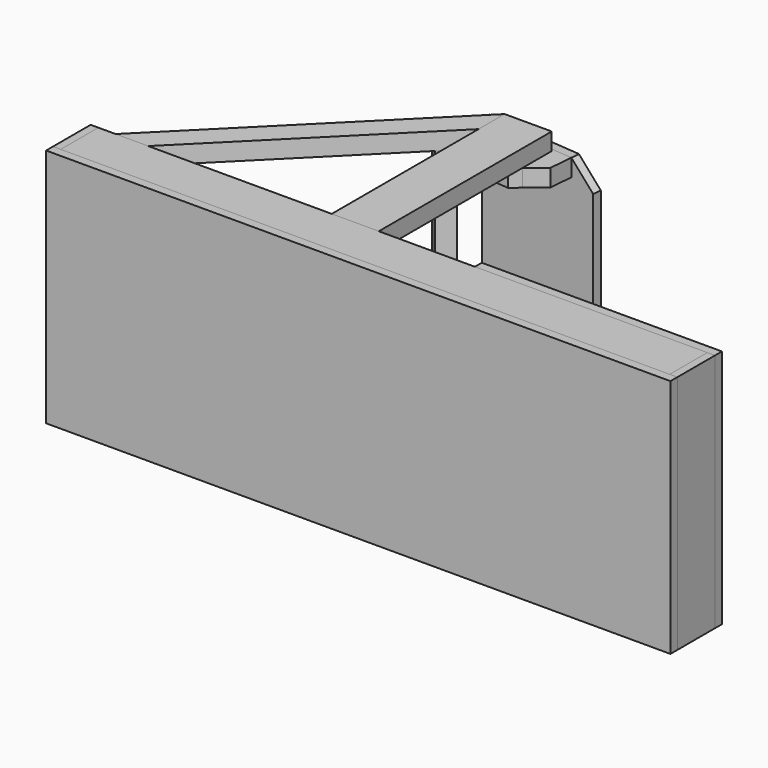
from build123d import *

# Parameters (mm, degrees)
F1_DEPTH       = 500
F2_DEPTH       = 36
F3_DEPTH       = 36
F4_DEPTH       = 36
F5_DEPTH       = 500
F0_W           = 16
F0_H           = 98
F6_DEPTH       = 500
F8_DEPTH       = 36
F9_DEPTH       = 428
F14_W          = 98
F14_H          = 428
F15_DEPTH      = 36
F16_W          = 98
F16_H          = 48
F17_DEPTH      = 36
F16_H_2        = 18
F18_DEPTH      = 104
F18_DEPTH_BACK = 36
F19_W          = 98
F19_H          = 36
F20_DEPTH      = 18
F22_DEPTH      = 36
F24_DEPTH      = 428
F26_DEPTH      = 18


with BuildPart() as f1:
    # F0 (on Top) → F1 (new body)
    with BuildSketch(Plane.XY):
        Polygon((1268, -98), (0, -98), (-16, -98), (-16, -116), (1284, -116), (1284, -98), align=None)
    extrude(amount=-F1_DEPTH)


with BuildPart() as f2:
    # F0 (on Top) → F2 (new body)
    with BuildSketch(Plane.XY):
        Polygon((36, 0), (0, 0), (0, -98), (1268, -98), (1268, 0), (784, 0), (584, 0), (486, 0), (103.8822509939, 0), align=None)
    extrude(amount=-F2_DEPTH)


with BuildPart() as f3:
    # F0 (on Top) → F3 (new body)
    with BuildSketch(Plane.XY):
        Polygon((584, 450), (486, 450), (486, 382.1177490061), (486, 0), (584, 0), align=None)
    extrude(amount=-F3_DEPTH)


with BuildPart() as f4:
    # F0 (on Top) → F4 (new body)
    with BuildSketch(Plane.XY):
        Polygon((486, 450), (36, 0), (103.8822509939, 0), (486, 382.1177490061), align=None)
    extrude(amount=-F4_DEPTH)


with BuildPart() as f5:
    # F0 (on Top) → F5 (new body)
    with BuildSketch(Plane.XY):
        Polygon((784, 0), (1268, 0), (1284, 0), (1284, 18), (784, 18), align=None)
    extrude(amount=-F5_DEPTH)


with BuildPart() as f6:
    # F0 (on Top) → F6 (new body)
    with BuildSketch(Plane.XY):
        with Locations((1276, -49)):
            Rectangle(F0_W, F0_H)
    extrude(amount=-F6_DEPTH)


with BuildPart() as f8:
    # F7 (on face) → F8 (new body)
    with BuildSketch(Plane(origin=(0, 0, -36), x_dir=(1, 0, 0), z_dir=(0, 0, -1))):
        Polygon((418.8753596794, -419.6689985812), (423.2171666194, -469.2960789942), (623.4523009358, -451.7777747019), (619.1816695412, -402.9642344955), (584, -373.4433085592), (584, -450), (486, -450), (486, -365.4289487301), (462.6759038301, -367.469542732), align=None)
        Polygon((566.0974979401, -358.4213256836), (486, -365.4289487301), (486, -450), (584, -450), (584, -373.4433085592), align=None)
    extrude(amount=F8_DEPTH)


with BuildPart() as f9:
    # F7 (on face) → F9 (new body)
    with BuildSketch(Plane(origin=(0, 0, -36), x_dir=(1, 0, 0), z_dir=(0, 0, -1))):
        Polygon((423.2171666194, -469.2960789942), (424.7859699888, -487.2275835599), (673.8346445118, -465.438647873), (672.2658411423, -447.5071433073), (623.4523009358, -451.7777747019), align=None)
    extrude(amount=F9_DEPTH)

    # F25 (on face) → F26 (cut, through all)
    with BuildSketch(Plane(origin=(43.9610143142, 502.4766928934, 0), x_dir=(0.9961946981, -0.0871557427, 0), z_dir=(-0.0871557427, -0.9961946981, 0))):
        Polygon((630.7048491943, -36), (581.7048491943, -36), (630.7048491943, -85), align=None)
        Polygon((630.7048491943, -464), (630.7048491943, -415), (581.7048491943, -464), align=None)
    extrude(amount=-F26_DEPTH, mode=Mode.SUBTRACT)


with BuildPart() as f11_1:
    # F11: instance of F3
    add(f3.part.mirror(Plane(origin=(317, -53.5, -250), x_dir=(1, 0, 0), z_dir=(0, 0, 1))))


with BuildPart() as f11_2:
    # F11: instance of F2
    add(f2.part.mirror(Plane(origin=(317, -53.5, -250), x_dir=(1, 0, 0), z_dir=(0, 0, 1))))


with BuildPart() as f11_3:
    # F11: instance of F4
    add(f4.part.mirror(Plane(origin=(317, -53.5, -250), x_dir=(1, 0, 0), z_dir=(0, 0, 1))))


with BuildPart() as f11_4:
    # F11: instance of F8
    add(f8.part.mirror(Plane(origin=(317, -53.5, -250), x_dir=(1, 0, 0), z_dir=(0, 0, 1))))


with BuildPart() as f13_1:
    # F13: instance of F6
    add(f6.part.mirror(Plane(origin=(634, -107, -250), x_dir=(0, -1, 0), z_dir=(-1, 0, 0))))


with BuildPart() as f15:
    # F14 (on face) → F15 (new body)
    with BuildSketch(Plane(origin=(784, 0, 0), x_dir=(0, -1, 0), z_dir=(-1, 0, 0))):
        with Locations((49, -250)):
            Rectangle(F14_W, F14_H)
    extrude(amount=-F15_DEPTH)


with BuildPart() as f17:
    # F16 (on face) → F17 (new body)
    with BuildSketch(Plane(origin=(0, 0, -500), x_dir=(1, 0, 0), z_dir=(0, 0, -1))):
        with Locations((535, -308)):
            Rectangle(F16_W, F16_H)
        Polygon((368, -332), (486, -332), (486, -284), (320, -284), align=None)
        Polygon((584, -284), (584, -332), (744, -332), (696, -284), align=None)
    extrude(amount=F17_DEPTH)


with BuildPart() as f18:
    # F16 (on face) → F18 (new body, two sides)
    with BuildSketch(Plane(origin=(0, 0, -500), x_dir=(1, 0, 0), z_dir=(0, 0, -1))) as f18_sk:
        Polygon((584, -332), (584, -350), (784, -350), (784, -332), (744, -332), align=None)
        with Locations((535, -341)):
            Rectangle(F16_W, F16_H_2)
    extrude(amount=F18_DEPTH)
    extrude(f18_sk.sketch, amount=-F18_DEPTH_BACK)

    # F19 (on face) → F20 (cut, through all)
    with BuildSketch(Plane(origin=(0, 350, 0), x_dir=(-1, 0, 0), z_dir=(0, 1, 0))):
        with Locations((-535, -482)):
            Rectangle(F19_W, F19_H)
        Polygon((-486, -604), (-486, -536), (-554, -604), align=None)
    extrude(amount=-F20_DEPTH, mode=Mode.SUBTRACT)


with BuildPart() as f22:
    # F21 (on face) → F22 (new body)
    with BuildSketch(Plane(origin=(0, 0, -500), x_dir=(1, 0, 0), z_dir=(0, 0, -1))):
        Polygon((851.8822509939, -18), (784, -18), (584, -218), (584, -285.8822509939), align=None)
    extrude(amount=-F22_DEPTH)


with BuildPart() as f24:
    # F23 (on face) → F24 (new body, through all)
    with BuildSketch(Plane.XY.offset(-464)):
        Polygon((461.3380951166, 357.4558441227), (427.3969696197, 391.3969696197), (401.941125497, 365.941125497), (435.8822509939, 332), align=None)
    extrude(amount=F24_DEPTH)


solid = Compound([f1.part, f2.part, f3.part, f4.part, f5.part, f6.part, f8.part, f9.part, f11_1.part, f11_2.part, f11_3.part, f11_4.part, f13_1.part, f15.part, f17.part, f18.part, f22.part, f24.part])
